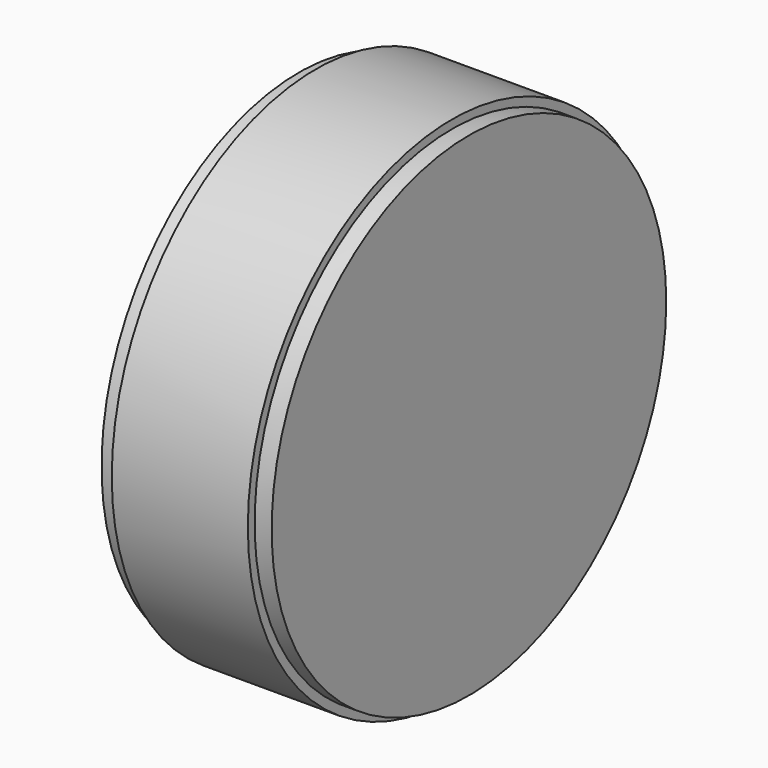
from build123d import *

# Parameters (mm, degrees)
F0_R     = 36.83
F1_DEPTH = 2.54
F2_R     = 38.1
F2_R_2   = 36.83
F3_DEPTH = 20.32
F4_R     = 36.83
F5_DEPTH = 2.54


with BuildPart() as f1:
    # F0 (on Right) → F1 (new body)
    with BuildSketch(Plane.YZ):
        Circle(F0_R)
    extrude(amount=-F1_DEPTH)

    # F2 (on face) → F3 (join)
    with BuildSketch(Plane.YZ):
        Circle(F2_R)
        Circle(F2_R_2, mode=Mode.SUBTRACT)
        Circle(F2_R_2)
    extrude(amount=F3_DEPTH)

    # F4 (on face) → F5 (join)
    with BuildSketch(Plane.YZ.offset(20.32)):
        Circle(F4_R)
    extrude(amount=F5_DEPTH)


solid = f1.part
